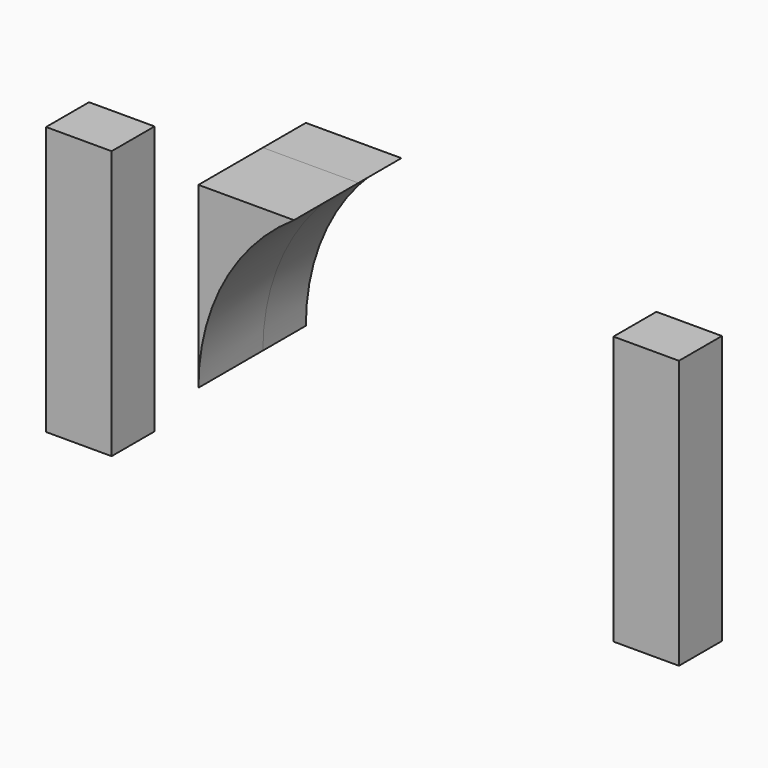
from build123d import *

# Parameters (mm, degrees)
F1_DEPTH = 10
F0_W     = 12.2
F0_H     = 50
F2_DEPTH = 15


with BuildPart() as f1:
    # F0 (on Front) → F1 (new body)
    with BuildSketch(Plane.XZ):
        with BuildLine():
            ThreePointArc((-18.5547723852, -8.2686455011), (-13.8274372079, 10.5950528717), (-0.7628165701, 25))
            Line((-0.7628165701, 25), (-18.5547723852, 25))
            Line((-18.5547723852, 25), (-18.5547723852, -8.2686455011))
        make_face()
    extrude(amount=F1_DEPTH)


with BuildPart() as f1b:
    # F0 (on Front) → F1, piece 2 (new body)
    with BuildSketch(Plane.XZ):
        with Locations((52.8224339074, -9.7424781105)):
            Rectangle(F0_W, F0_H)
    extrude(amount=F1_DEPTH)


with BuildPart() as f1c:
    # F0 (on Front) → F1, piece 3 (new body)
    with BuildSketch(Plane.XZ):
        with Locations((-52.8224339074, -9.7424781105)):
            Rectangle(F0_W, F0_H)
    extrude(amount=F1_DEPTH)


with BuildPart() as f2:
    # F2 (new): a face of the model
    f2_faces = [f1.part.faces().sort_by_distance(p)[0] for p in [
        (-13.5079798624, -10, 17.0974885768),
    ]]
    extrude(f2_faces, amount=F2_DEPTH)


solid = Compound([f1.part, f1b.part, f1c.part, f2.part])
